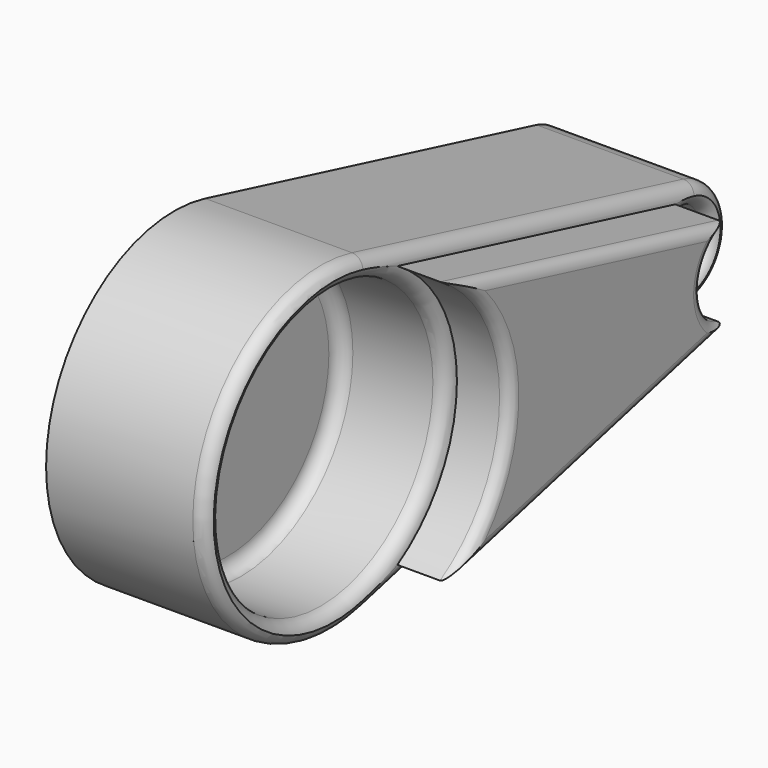
from build123d import *

# Parameters (mm, degrees)
F1_DEPTH = 76.2
F2_R     = 15.875
F2_R_2   = 66.675
F3_DEPTH = 50.8
F4_F1_R  = 6.35
F4_F2_R  = 6.35
F4_F3_R  = 6.35
F5_T     = -2.54
F6_DEPTH = 25.4
F7_R     = 5.08


# Not quite as in the source:
# - a fillet or chamfer that OpenCascade refuses, or shapes differently, is made with other operations: its cross-section is extruded or revolved along the edge and cut away or added


with BuildPart() as f1:
    # F0 (on Right) → F1 (new body)
    with BuildSketch(Plane.YZ):
        with BuildLine():
            ThreePointArc((18.4812146278, -73.9248585111), (60.0612543768, -46.8944103565), (76.2, 0))
            ThreePointArc((76.2, 0), (60.0612543768, 46.8944103565), (18.4812146278, 73.9248585111))
            ThreePointArc((18.4812146278, 73.9248585111), (-76.2, 0), (18.4812146278, -73.9248585111))
        make_face()
        with BuildLine():
            ThreePointArc((18.4812146278, 73.9248585111), (60.0612543768, 46.8944103565), (76.2, 0))
            ThreePointArc((76.2, 0), (60.0612543768, -46.8944103565), (18.4812146278, -73.9248585111))
            Line((18.4812146278, -73.9248585111), (215.6141706573, -24.6416195037))
            ThreePointArc((215.6141706573, -24.6416195037), (184.0537657814, 0), (215.6141706573, 24.6416195037))
            Line((215.6141706573, 24.6416195037), (18.4812146278, 73.9248585111))
        make_face()
        with BuildLine():
            ThreePointArc((234.8537657814, 0), (229.474183907, 15.6314701188), (215.6141706573, 24.6416195037))
            ThreePointArc((215.6141706573, 24.6416195037), (184.0537657814, 0), (215.6141706573, -24.6416195037))
            ThreePointArc((215.6141706573, -24.6416195037), (229.474183907, -15.6314701188), (234.8537657814, 0))
        make_face()
    extrude(amount=F1_DEPTH)

    # F2 (on face) → F3 (cut)
    with BuildSketch(Plane.YZ.offset(76.2)):
        with Locations((209.4537657814, 0)):
            Circle(F2_R)
        Circle(F2_R_2)
    extrude(amount=-F3_DEPTH, mode=Mode.SUBTRACT)

    # F4: fillet of radius 6.35 on 8 edges, made by hand

    # F4_f1
    f4_f1_edges = [f1.edges().sort_by_distance(p)[0] for p in [
        (76.2, -76.2, 0),
        (76.2, 117.0476926425, 49.2832390074),
        (76.2, 117.0476926425, -49.2832390074),
        (76.2, 234.8537657814, 0),
    ]]
    fillet(f4_f1_edges, radius=F4_F1_R)

    # F4_f2
    f4_f2_edges = [f1.edges().sort_by_distance(p)[0] for p in [
        (25.4, -66.675, 0),
    ]]
    fillet(f4_f2_edges, radius=F4_F2_R)

    # F4_f3
    f4_f3_edges = [f1.edges().sort_by_distance(p)[0] for p in [
        (25.4, 193.5787657814, 0),
    ]]
    fillet(f4_f3_edges, radius=F4_F3_R)

    # F4_s4 → F4_t5 (revolve, cut)
    with BuildSketch(Plane.XY):
        with BuildLine():
            ThreePointArc((76.2, 73.025), (74.3401280605, 68.5348719395), (69.85, 66.675))
            Line((69.85, 66.675), (69.85, 66.548))
            Line((69.85, 66.548), (76.327, 66.548))
            Line((76.327, 66.548), (76.327, 73.025))
            Line((76.327, 73.025), (76.2, 73.025))
        make_face()
    revolve(axis=Axis((76.2, 0, 0), (1, 0, 0)), mode=Mode.SUBTRACT)

    # F4_s6 → F4_t7 (revolve, cut)
    with BuildSketch(Plane.XY):
        with BuildLine():
            ThreePointArc((69.85, 225.3287657814), (74.3401280605, 227.1886377208), (76.2, 231.6787657814))
            Line((76.2, 231.6787657814), (76.327, 231.6787657814))
            Line((76.327, 231.6787657814), (76.327, 225.2017657814))
            Line((76.327, 225.2017657814), (69.85, 225.2017657814))
            Line((69.85, 225.2017657814), (69.85, 225.3287657814))
        make_face()
    revolve(axis=Axis((76.2, 209.4537657814, 0), (1, 0, 0)), mode=Mode.SUBTRACT)

    # F5
    f5_openings = [f1.faces().sort_by_distance(p)[0] for p in [
        (0, 57.51924, 0),
    ]]
    offset(amount=F5_T, openings=f5_openings)

    # F6 (add): a face of the model
    f6_faces = [f1.faces().sort_by_distance(p)[0] for p in [
        (76.2, 119.1189366743, 0),
    ]]
    extrude(f6_faces, amount=F6_DEPTH)

    # F7
    f7_edges = [f1.edges().sort_by_distance(p)[0] for p in [
        (101.6, 187.228766, 0),
        (101.6, 120.285991, 41.928234),
        (101.6, 73.025, 0),
        (101.6, 120.285991, -41.928234),
    ]]
    fillet(f7_edges, radius=F7_R)


solid = f1.part
